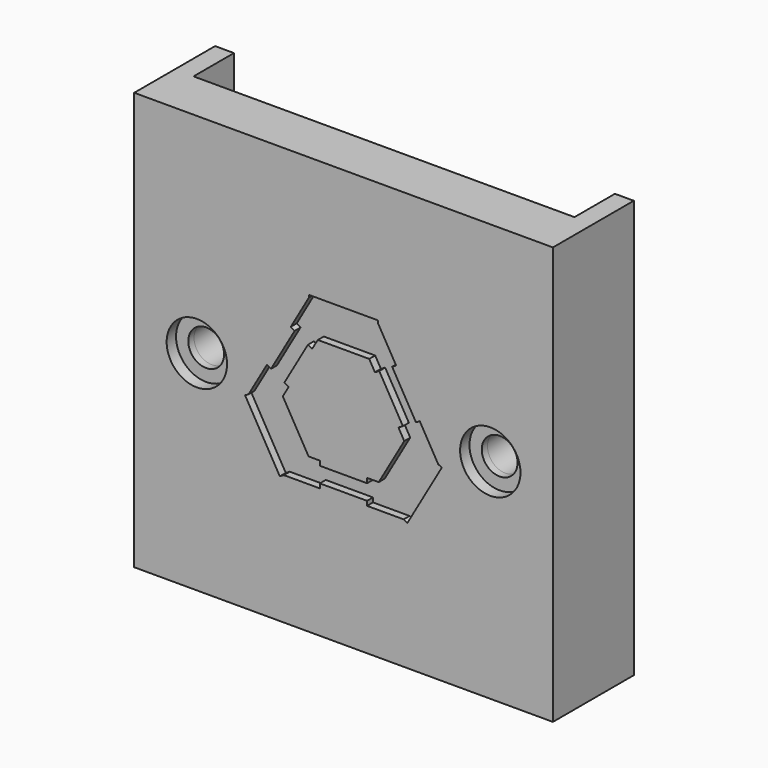
from build123d import *
from build123d import SkipClean  # not in build123d's __all__

# Parameters (mm, degrees)
F1_DEPTH      = 24.13
F2_R          = 2.032
F2_R_2        = 1.2065
F3_DEPTH      = 0.7874
F4_DEPTH      = 25.4
F6_DEPTH      = 0.5
F7_DEPTH      = 2
F8_DEPTH      = 2
F9_W          = 25.654
F9_H          = 1
F10_DEPTH     = 1.27
F11_R         = 1.2065
F12_DEPTH     = 1.905
F13_DEPTH     = 1.905
F14_DEPTH     = 1.0414
F15_TEXT_SIZE = 7.0384462024
F16_DEPTH     = 0.5588


# Not quite as in the source:
# - after a boolean that leaves OpenCascade's solid faulty, fix() repairs it
# - a feature names something its author has since deleted; it is built from what else it names
# - Text() gives the source's letters only with a copy of the font that has no kerning and outlines rounded to 1/6400 em; it was checked with that copy


with BuildPart() as f1:
    # F0 (on Top) → F1 (new body)
    with BuildSketch(Plane.XY):
        Polygon((-22.881621525, -1.6067087497), (-22.881621525, 2.0254912503), (-24.151621525, 2.0254912503), (-24.151621525, -2.8767087497), (4.042378475, -2.8767087497), (4.042378475, 2.0254912503), (2.772378475, 2.0254912503), (2.772378475, -1.6067087497), align=None)
    extrude(amount=F1_DEPTH)

    # F2 (on face) → F3 (cut)
    with BuildSketch(Plane.XZ.offset(2.8767087497)):
        with Locations((-19.935221525, 12.065)):
            Circle(F2_R)
        with Locations((-19.935221525, 12.065)):
            Circle(F2_R_2, mode=Mode.SUBTRACT)
        with Locations((-0.174021525, 12.065)):
            Circle(F2_R)
        with Locations((-0.174021525, 12.065)):
            Circle(F2_R_2, mode=Mode.SUBTRACT)
    extrude(amount=-F3_DEPTH, mode=Mode.SUBTRACT)

    # F4 (cut): faces of the model
    f4_faces = [f1.faces().sort_by_distance(p)[0] for p in [
        (-19.935221525, -2.8767087497, 12.065),
        (-0.174021525, -2.8767087497, 12.065),
    ]]
    extrude(f4_faces, amount=-F4_DEPTH, mode=Mode.SUBTRACT)

    # F5 (on face) → F6 (cut)
    with BuildSketch(Plane.XZ.offset(2.8767087497)):
        Polygon((-12.3912415756, 17.8113617003), (-13.6065593278, 15.684556216), (-13.3501001609, 15.5277705701), (-14.9427792273, 12.7550959473), (-15.21558023, 12.9117982314), (-16.4524054843, 10.7586249602), (-16.6849697297, 10.6241926551), (-14.3470017528, 6.5795714036), (-14.0742704561, 6.7396221901), (-11.6537952153, 6.7396221901), (-11.6537952153, 7.0368205197), (-8.471750264, 7.0368205197), (-8.471750264, 6.7396221901), (-6.0077723583, 6.7396221901), (-5.7620638571, 6.5984823741), (-3.4414858846, 10.6383468956), (-3.6771140247, 10.7619399543), (-4.9225916905, 12.9113931759), (-5.1792576933, 12.7626708074), (-6.7848130465, 15.533548376), (-6.5128039159, 15.6911611557), (-7.7413314311, 17.8113617003), (-7.7413314311, 17.9749652743), (-12.3912415756, 17.9749652743), align=None)
        Polygon((-12.1788967651, 14.8354667667), (-11.7852579159, 15.4973436147), (-8.3281154101, 15.4973436147), (-7.9414616069, 14.830054039), (-7.6521674377, 14.9976824493), (-6.0583813106, 12.2471162856), (-6.3580625964, 12.0734691718), (-5.9656283895, 11.396203739), (-7.6865507823, 8.4002719491), (-8.471750264, 8.4002719491), (-8.471750264, 8.0795111135), (-11.6385354949, 8.0795111135), (-11.6385354949, 8.3887251094), (-12.4105562744, 8.3887251094), (-14.1476861274, 11.3866747806), (-13.7563398992, 12.0679644255), (-14.0430930461, 12.2326810967), (-12.4564279131, 14.9948861397), align=None, mode=Mode.SUBTRACT)
    extrude(amount=-F6_DEPTH, mode=Mode.SUBTRACT)

    # F7 (add): a face of the model
    f7_faces = [f1.faces().sort_by_distance(p)[0] for p in [
        (-10.054621525, -1.7395492941, 0),
    ]]
    extrude(f7_faces, amount=F7_DEPTH)

    # F8 (add): a face of the model
    f8_faces = [f1.faces().sort_by_distance(p)[0] for p in [
        (-10.054621525, -1.7395492941, 24.13),
    ]]
    extrude(f8_faces, amount=F8_DEPTH)

    # F9 (on face) → F10 (join)
    with BuildSketch(Plane(origin=(0, -1.6067087497, 0), x_dir=(-1, 0, 0), z_dir=(0, 1, 0))):
        with Locations((10.054621525, 25.63)):
            Rectangle(F9_W, F9_H)
        with Locations((10.054621525, -1.5)):
            Rectangle(F9_W, F9_H)
    extrude(amount=F10_DEPTH)

    # F11 (on face) → F12 (join)
    with BuildSketch(Plane(origin=(0, -1.6067087497, 0), x_dir=(-1, 0, 0), z_dir=(0, 1, 0))):
        with BuildLine():
            ThreePointArc((-2.772378475, 6.4958446701), (-1.4028429606, 8.7376625106), (0.8266095876, 10.1272365784))
            ThreePointArc((0.8266095876, 10.1272365784), (2.218721566, 12.065), (0.8266095876, 14.0027634216))
            ThreePointArc((0.8266095876, 14.0027634216), (-1.4028429606, 15.3923374894), (-2.772378475, 17.6341553299))
            Line((-2.772378475, 17.6341553299), (-2.772378475, 6.4958446701))
        make_face()
        with Locations((0.174021525, 12.065)):
            Circle(F11_R, mode=Mode.SUBTRACT)
        with BuildLine():
            ThreePointArc((19.2826334624, 10.1272365784), (21.5120860106, 8.7376625106), (22.881621525, 6.4958446701))
            Line((22.881621525, 6.4958446701), (22.881621525, 17.6341553299))
            ThreePointArc((22.881621525, 17.6341553299), (21.5120860106, 15.3923374894), (19.2826334624, 14.0027634216))
            ThreePointArc((19.2826334624, 14.0027634216), (17.890521484, 12.065), (19.2826334624, 10.1272365784))
        make_face()
        with Locations((19.935221525, 12.065)):
            Circle(F11_R, mode=Mode.SUBTRACT)
    with SkipClean():  # cleaning this boolean's faces spoils the solid; the shape is the same uncleaned
        extrude(amount=F12_DEPTH)

    # F13 (add): faces of the model
    f13_faces = [f1.faces().sort_by_distance(p)[0] for p in [
        (-23.516621525, 2.0254912503, 12.065),
        (-10.054621525, -0.3367087497, 25.63),
        (-10.054621525, -0.3367087497, -1.5),
        (3.407378475, 2.0254912503, 12.065),
    ]]
    extrude(f13_faces, amount=F13_DEPTH)

    add(f1.part.fix(), mode=Mode.REPLACE)

    # F14 (cut): a face of the model
    f14_faces = [f1.faces().sort_by_distance(p)[0] for p in [
        (-10.054621525, 1.5682912503, 25.63),
    ]]
    extrude(f14_faces, amount=-F14_DEPTH, mode=Mode.SUBTRACT)

    # F15 (on face) → F16 (cut)
    with BuildSketch(Plane(origin=(0, -1.6067087497, 0), x_dir=(-1, 0, 0), z_dir=(0, 1, 0))):
        with Locations((-2.772378475, -1)):
            Text('2/6/17', F15_TEXT_SIZE, font='Open Sans', text_align=(TextAlign.LEFT, TextAlign.BOTTOM))
    extrude(amount=-F16_DEPTH, mode=Mode.SUBTRACT)


solid = f1.part
